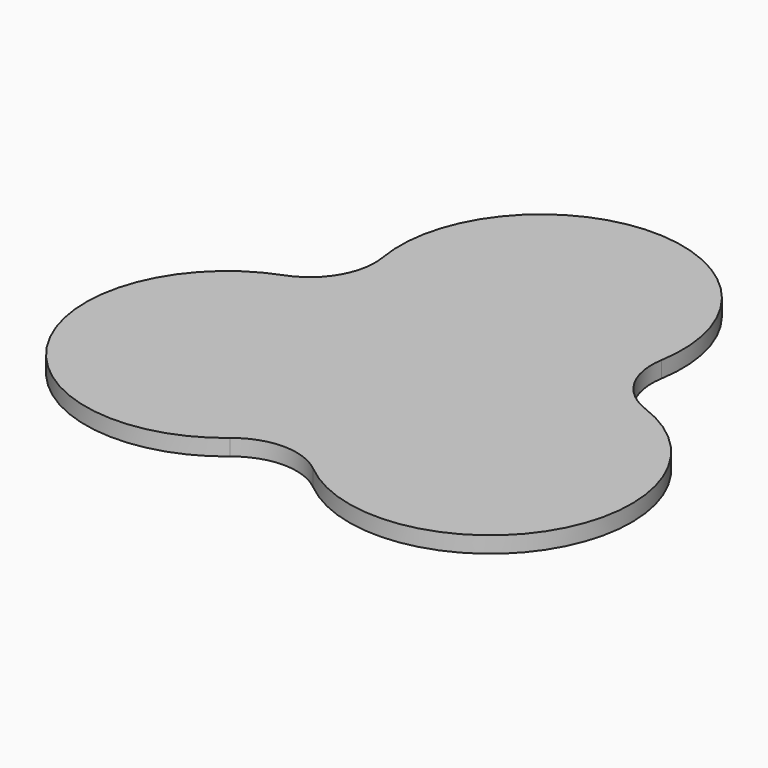
from build123d import *

# Parameters (mm, degrees)
F1_DEPTH = 3


# Not quite as in the source:
# - ends of sketch curves that miss each other by under 0.0002 mm in the source are joined


with BuildPart() as f1:
    # F0 (on Top) → F1 (new body)
    with BuildSketch(Plane.XY):
        with BuildLine():
            ThreePointArc((32.9074971055, 11.248177677), (26.6878329895, 16.4993586176), (25.2500089531, 24.5113362153))
            ThreePointArc((25.2500089531, 24.5113362153), (-0.3819362324, 54.8706200704), (-26.0138819919, 24.5113361177))
            ThreePointArc((-26.0138819919, 24.5113361177), (-27.4517054543, 16.4993586176), (-33.6713695703, 11.248177677))
            ThreePointArc((-33.6713695703, 11.248177677), (-47.1473080368, -26.1293799296), (-8.0394240132, -33.1476541294))
            ThreePointArc((-8.0394240132, -33.1476541294), (-0.3819362324, -30.3868579581), (7.2755513239, -33.1476544003))
            ThreePointArc((7.2755513239, -33.1476544003), (46.383435572, -26.1293799296), (32.9074971055, 11.248177677))
        make_face()
    extrude(amount=-F1_DEPTH)


solid = f1.part
